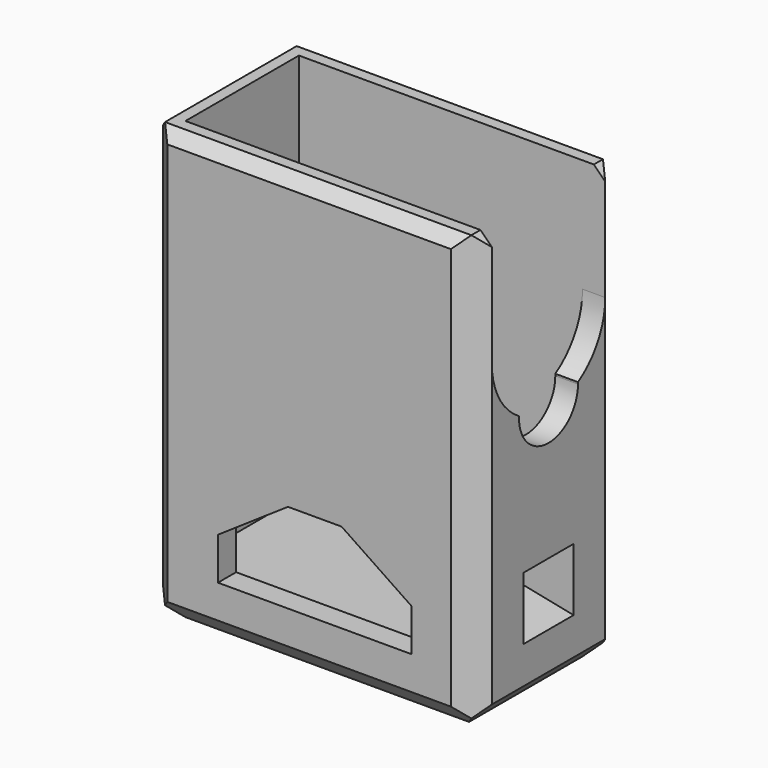
from build123d import *

# Parameters (mm, degrees)
F0_W      = 29
F0_H      = 16.5
F1_DEPTH  = 38.5
F2_T      = -2
F3_DEPTH  = 2.25
F4_SIZE   = 2
F5_SIZE   = 2
F6_SIZE   = 0.99999
F8_DEPTH  = 16.501
F9_W      = 12.5
F9_H      = 0.99999
F10_DEPTH = 2
F11_R     = 2
F12_DEPTH = 2.001
F13_W     = 7.54
F13_H     = 7.25
F13_R     = 1.1
F14_DEPTH = 4.35
F15_W     = 5.538
F15_H     = 5.533
F17_W     = 5.481
F17_H     = 4.583


# Not quite as in the source:
# - a fillet or chamfer is up to 0.001 mm smaller than in the source, because OpenCascade refuses the exact size


with BuildPart() as f1:
    # F0 (on Top) → F1 (new body)
    with BuildSketch(Plane.XY):
        with Locations((14.5, 8.25)):
            Rectangle(F0_W, F0_H)
    extrude(amount=F1_DEPTH)

    # F2
    f2_openings = [f1.faces().sort_by_distance(p)[0] for p in [
        (14.5, 8.25, 38.5),
    ]]
    offset(amount=F2_T, openings=f2_openings)

    # F3 (add): a face of the model
    f3_faces = [f1.faces().sort_by_distance(p)[0] for p in [
        (14.5, 8.25, 2),
    ]]
    extrude(f3_faces, amount=F3_DEPTH)

    # F4
    f4_edges = [f1.edges().sort_by_distance(p)[0] for p in [
        (0, 0, 19.25),
        (29, 0, 19.25),
        (29, 16.5, 19.25),
        (0, 16.5, 19.25),
    ]]
    chamfer(f4_edges, length=F4_SIZE)

    # F5 (call 1 of 4: OpenCascade refuses the feature's edges together)
    f5_edges = [f1.edges().sort_by_distance(p)[0] for p in [
        (14.5, 0, 0),
    ]]
    chamfer(f5_edges, length=F5_SIZE)

    # F5#2 (call 2 of 4)
    f5_2_edges = [f1.edges().sort_by_distance(p)[0] for p in [
        (0, 8.25, 0),
    ]]
    chamfer(f5_2_edges, length=F5_SIZE)

    # F5#3 (call 3 of 4)
    f5_3_edges = [f1.edges().sort_by_distance(p)[0] for p in [
        (14.5, 16.5, 0),
    ]]
    chamfer(f5_3_edges, length=F5_SIZE)

    # F5#4 (call 4 of 4)
    f5_4_edges = [f1.edges().sort_by_distance(p)[0] for p in [
        (29, 8.25, 0),
    ]]
    chamfer(f5_4_edges, length=F5_SIZE)

    # F6 (size 1 in the source; OpenCascade refuses exactly that, so slightly less here)
    f6_edges = [f1.edges().sort_by_distance(p)[0] for p in [
        (0, 8.25, 38.5),
        (14.5, 16.5, 38.5),
        (29, 8.25, 38.5),
        (14.5, 0, 38.5),
    ]]
    chamfer(f6_edges, length=F6_SIZE)

    # F7 (on face) → F8 (cut, through all)
    with BuildSketch(Plane.XZ):
        Polygon((6.464, 8.664), (6.464, 4.94), (23.536, 4.94), (23.536, 8.664), (17.364, 12.834), (12.635, 12.834), align=None)
    extrude(amount=-F8_DEPTH, mode=Mode.SUBTRACT)

    # F9 (on face) → F10 (cut, through all)
    with BuildSketch(Plane.YZ.offset(29)):
        with BuildLine():
            ThreePointArc((5.0038961688, 23.1590909091), (8.25, 22.25), (11.4961038312, 23.1590909091))
            ThreePointArc((11.4961038312, 23.1590909091), (8.25, 26.25), (5.0038961688, 23.1590909091))
        make_face()
        with BuildLine():
            ThreePointArc((5.0038961688, 23.1590909091), (8.1704306945, 19.7509741882), (11.5, 23))
            ThreePointArc((11.5, 23), (11.4990258118, 23.0795693055), (11.4961038312, 23.1590909091))
            ThreePointArc((11.4961038312, 23.1590909091), (8.25, 22.25), (5.0038961688, 23.1590909091))
        make_face()
        with BuildLine():
            ThreePointArc((5.0038961688, 23.1590909091), (8.25, 26.25), (11.4961038312, 23.1590909091))
            ThreePointArc((11.4961038312, 23.1590909091), (13.6975062618, 25.4361502113), (14.5, 28.5))
            Line((14.5, 28.5), (2, 28.5))
            ThreePointArc((2, 28.5), (2.8024937382, 25.4361502113), (5.0038961688, 23.1590909091))
        make_face()
        with BuildLine():
            Line((2, 28.5), (14.5, 28.5))
            ThreePointArc((14.5, 28.5), (8.25, 34.75), (2, 28.5))
        make_face()
        with BuildLine():
            ThreePointArc((2, 28.5), (8.25, 34.75), (14.5, 28.5))
            Line((14.5, 28.5), (14.5, 37.50001))
            Line((14.5, 37.50001), (2, 37.50001))
            Line((2, 37.50001), (2, 28.5))
        make_face()
        with Locations((8.25, 38.000005)):
            Rectangle(F9_W, F9_H)
    extrude(amount=-F10_DEPTH, mode=Mode.SUBTRACT)

    # F11 (on face) → F12 (cut, through all)
    with BuildSketch(Plane.YZ.offset(2)):
        with Locations((8.25, 23)):
            Circle(F11_R)
    extrude(amount=-F12_DEPTH, mode=Mode.SUBTRACT)

    # F13 (on face) → F14 (join)
    with BuildSketch(Plane(origin=(27, 0, 0), x_dir=(0, -1, 0), z_dir=(-1, 0, 0))):
        with Locations((-8.25, 7.875)):
            Rectangle(F13_W, F13_H)
        with Locations((-8.25, 9)):
            Circle(F13_R, mode=Mode.SUBTRACT)
    extrude(amount=F14_DEPTH)

    # F15 (on face) → F18 section 0
    with BuildSketch(Plane.YZ.offset(29)):
        with Locations((8.25, 8.0385)):
            Rectangle(F15_W, F15_H)
    # F17 (on offset) → F18 section 1
    with BuildSketch(Plane.YZ.offset(24.55)):
        with Locations((8.2215, 8.5135)):
            Rectangle(F17_W, F17_H)
    loft(mode=Mode.SUBTRACT)


solid = f1.part
